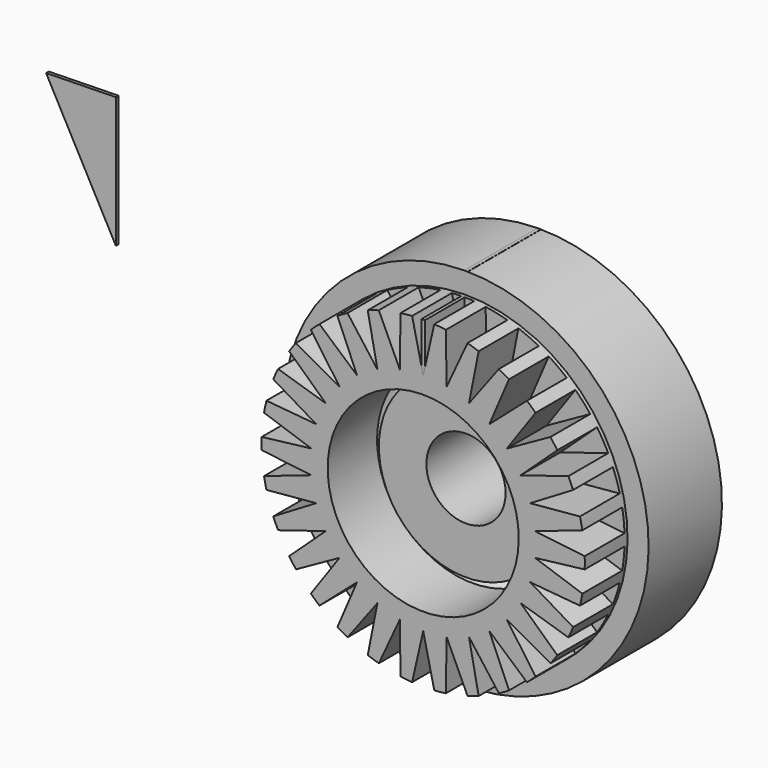
from build123d import *

# Parameters (mm, degrees)
F2_DEPTH = 0.5
F0_W     = 16.1312930286
F0_H     = 19.9230848044
F5_DEPTH = 15
F7_DEPTH = 1


with BuildPart() as f2:
    # F0 (on Right) → F2 (new body, symmetric)
    with BuildSketch(Plane.YZ):
        with BuildLine():
            Line((0, 16.1320931972), (0, 11.9378846139))
            Line((0, 11.9378846139), (13.8204824179, 11.9378846139))
            Line((13.8204824179, 11.9378846139), (13.8204824179, 26.2730848044))
            Line((13.8204824179, 26.2730848044), (11.3400983003, 26.2730848044))
            ThreePointArc((11.3400983003, 26.2730848044), (7.6065356805, 19.0371254581), (0, 16.1320931972))
        make_face()
        with BuildLine():
            Line((-13.8204824179, 11.9378846139), (0, 11.9378846139))
            Line((0, 11.9378846139), (0, 16.1320931972))
            ThreePointArc((0, 16.1320931972), (-7.6065356805, 19.0371254581), (-11.3400983003, 26.2730848044))
            Line((-11.3400983003, 26.2730848044), (-13.8204824179, 26.2730848044))
            Line((-13.8204824179, 26.2730848044), (-13.8204824179, 11.9378846139))
        make_face()
    extrude(amount=F2_DEPTH, both=True)


with BuildPart() as f2b:
    # F0 (on Right) → F2, piece 2 (new body, symmetric)
    with BuildSketch(Plane.YZ):
        with Locations((-21.8861289322, 38.7746272066)):
            Rectangle(F0_W, F0_H)
        with BuildLine():
            Line((-13.8204824179, 28.8130848044), (-11.3400983003, 28.8130848044))
            ThreePointArc((-11.3400983003, 28.8130848044), (0, 38.9540764116), (11.3400983003, 28.8130848044))
            Line((11.3400983003, 28.8130848044), (13.8204824179, 28.8130848044))
            Line((13.8204824179, 28.8130848044), (13.8204824179, 55.0861696088))
            Line((13.8204824179, 55.0861696088), (0, 55.0861696088))
            Line((0, 55.0861696088), (-13.8204824179, 55.0861696088))
            Line((-13.8204824179, 55.0861696088), (-13.8204824179, 48.7361696088))
            Line((-13.8204824179, 48.7361696088), (-13.8204824179, 28.8130848044))
        make_face()
    extrude(amount=F2_DEPTH, both=True)


with BuildPart() as f3:
    # F2_face (on face) → F3 (revolve)
    with BuildSketch(Plane(origin=(-0.5, -8.0664830441, 42.5658458946), x_dir=(0, 1, 0), z_dir=(-1, 0, 0))):
        with BuildLine():
            Line((-21.8852924024, -6.1703237142), (-5.7539993738, -6.1703237142))
            Line((-5.7539993738, -6.1703237142), (-5.7539993738, -12.5203237142))
            Line((-5.7539993738, -12.5203237142), (21.8869654621, -12.5203237142))
            Line((21.8869654621, -12.5203237142), (21.8869654621, 13.7527610902))
            Line((21.8869654621, 13.7527610902), (19.4065813444, 13.7527610902))
            ThreePointArc((19.4065813444, 13.7527610902), (8.0664830441, 3.611769483), (-3.2736152561, 13.7527610902))
            Line((-3.2736152561, 13.7527610902), (-21.8852924024, 13.7527610902))
            Line((-21.8852924024, 13.7527610902), (-21.8852924024, -6.1703237142))
        make_face()
    revolve(axis=Axis((0, -0.1056473702, 0), (0, -1, 0)))

    # F4 (on face) → F5 (cut)
    with BuildSketch(Plane.XZ.offset(29.9517754465)):
        with BuildLine():
            Line((-7.0547712791, 33.1900893753), (-6.8376785657, 48.2567133151))
            ThreePointArc((-6.8376785657, 48.2567133151), (-8.490521681, 47.9934919518), (-10.1333526715, 47.6736760883))
            ThreePointArc((-10.1333526715, 47.6736760883), (-11.7642342913, 47.2976428554), (-13.3812433852, 46.865835676))
            Line((-13.3812433852, 46.865835676), (-7.0547712791, 33.1900893753))
        make_face()
        with BuildLine():
            ThreePointArc((3.3448759751, 48.6238216603), (1.6734246487, 48.7099977221), (0, 48.7387343716))
            ThreePointArc((0, 48.7387343716), (-1.6734246487, 48.7099977221), (-3.3448759751, 48.6238216603))
            Line((-3.3448759751, 48.6238216603), (0, 33.9315757155))
            Line((0, 33.9315757155), (3.3448759751, 48.6238216603))
        make_face()
        with BuildLine():
            ThreePointArc((10.1333526715, 47.6736760883), (8.490521681, 47.9934919518), (6.8376785657, 48.2567133151))
            Line((6.8376785657, 48.2567133151), (7.0547712791, 33.1900893753))
            Line((7.0547712791, 33.1900893753), (13.3812433852, 46.865835676))
            ThreePointArc((13.3812433852, 46.865835676), (11.7642342913, 47.2976428554), (10.1333526715, 47.6736760883))
        make_face()
        with BuildLine():
            ThreePointArc((19.823829206, 44.5250493964), (18.2833914712, 45.1794402849), (16.7213937422, 45.7805550366))
            Line((16.7213937422, 45.7805550366), (13.8012152008, 30.9980368656))
            Line((13.8012152008, 30.9980368656), (22.832786249, 43.0595877854))
            ThreePointArc((22.832786249, 43.0595877854), (21.3408904443, 43.8181540367), (19.823829206, 44.5250493964))
        make_face()
        with BuildLine():
            ThreePointArc((28.647909279, 39.4304643909), (27.2771893206, 40.3908302825), (25.8743037741, 41.3035668235))
            Line((25.8743037741, 41.3035668235), (19.9444797926, 27.4512213998))
            Line((19.9444797926, 27.4512213998), (31.2864267899, 37.3714292858))
            ThreePointArc((31.2864267899, 37.3714292858), (29.9848472799, 38.4236016238), (28.647909279, 39.4304643909))
        make_face()
        with BuildLine():
            ThreePointArc((36.2199382485, 32.6125788832), (35.0788431063, 33.83694718), (33.8963825724, 35.0214145438))
            Line((33.8963825724, 35.0214145438), (25.2160749133, 22.7046558333))
            Line((25.2160749133, 22.7046558333), (38.3727003512, 30.0499599983))
            ThreePointArc((38.3727003512, 30.0499599983), (37.3183224061, 31.349753443), (36.2199382485, 32.6125788832))
        make_face()
        with BuildLine():
            ThreePointArc((42.2089821141, 24.3693671858), (41.3473831213, 25.8042271182), (40.4370267994, 27.2086583971))
            Line((40.4370267994, 27.2086583971), (29.3856065601, 16.9657878578))
            Line((29.3856065601, 16.9657878578), (43.7819027744, 21.4151632632))
            ThreePointArc((43.7819027744, 21.4151632632), (43.02080777, 22.9057706039), (42.2089821141, 24.3693671858))
        make_face()
        with BuildLine():
            ThreePointArc((46.35329092, 15.0610972051), (45.8088440871, 16.6437385088), (45.2103789168, 18.2067533168))
            Line((45.2103789168, 18.2067533168), (32.2708461924, 10.485433542))
            Line((32.2708461924, 10.485433542), (47.2776259576, 11.8444211322))
            ThreePointArc((47.2776259576, 11.8444211322), (46.8430773976, 13.4606956754), (46.35329092, 15.0610972051))
        make_face()
        with BuildLine():
            ThreePointArc((48.471738485, 5.0945850055), (48.268238751, 6.7558386611), (48.0078205322, 8.4091257508))
            Line((48.0078205322, 8.4091257508), (33.7456949935, 3.5468154658))
            Line((33.7456949935, 3.5468154658), (48.7070900231, 1.7560209619))
            ThreePointArc((48.7070900231, 1.7560209619), (48.6180797649, 3.4273237543), (48.471738485, 5.0945850055))
        make_face()
        with BuildLine():
            ThreePointArc((48.471738485, -5.0945850055), (48.6180797649, -3.4273237543), (48.7070900231, -1.7560209619))
            Line((48.7070900231, -1.7560209619), (33.7456949935, -3.5468154658))
            Line((33.7456949935, -3.5468154658), (48.0078205322, -8.4091257508))
            ThreePointArc((48.0078205322, -8.4091257508), (48.268238751, -6.7558386611), (48.471738485, -5.0945850055))
        make_face()
        with BuildLine():
            ThreePointArc((46.35329092, -15.0610972051), (46.8430773976, -13.4606956754), (47.2776259576, -11.8444211322))
            Line((47.2776259576, -11.8444211322), (32.2708461924, -10.485433542))
            Line((32.2708461924, -10.485433542), (45.2103789168, -18.2067533168))
            ThreePointArc((45.2103789168, -18.2067533168), (45.8088440871, -16.6437385088), (46.35329092, -15.0610972051))
        make_face()
        with BuildLine():
            ThreePointArc((42.2089821141, -24.3693671858), (43.02080777, -22.9057706039), (43.7819027744, -21.4151632632))
            Line((43.7819027744, -21.4151632632), (29.3856065601, -16.9657878578))
            Line((29.3856065601, -16.9657878578), (40.4370267994, -27.2086583971))
            ThreePointArc((40.4370267994, -27.2086583971), (41.3473831213, -25.8042271182), (42.2089821141, -24.3693671858))
        make_face()
        with BuildLine():
            ThreePointArc((36.2199382485, -32.6125788832), (37.3183224061, -31.349753443), (38.3727003512, -30.0499599983))
            Line((38.3727003512, -30.0499599983), (25.2160749133, -22.7046558333))
            Line((25.2160749133, -22.7046558333), (33.8963825724, -35.0214145438))
            ThreePointArc((33.8963825724, -35.0214145438), (35.0788431063, -33.83694718), (36.2199382485, -32.6125788832))
        make_face()
        with BuildLine():
            ThreePointArc((28.647909279, -39.4304643909), (29.9848472799, -38.4236016238), (31.2864267899, -37.3714292858))
            Line((31.2864267899, -37.3714292858), (19.9444797926, -27.4512213998))
            Line((19.9444797926, -27.4512213998), (25.8743037741, -41.3035668235))
            ThreePointArc((25.8743037741, -41.3035668235), (27.2771893206, -40.3908302825), (28.647909279, -39.4304643909))
        make_face()
        with BuildLine():
            ThreePointArc((19.823829206, -44.5250493964), (21.3408904443, -43.8181540367), (22.832786249, -43.0595877854))
            Line((22.832786249, -43.0595877854), (13.8012152008, -30.9980368656))
            Line((13.8012152008, -30.9980368656), (16.7213937422, -45.7805550366))
            ThreePointArc((16.7213937422, -45.7805550366), (18.2833914712, -45.1794402849), (19.823829206, -44.5250493964))
        make_face()
        with BuildLine():
            ThreePointArc((10.1333526715, -47.6736760883), (11.7642342913, -47.2976428554), (13.3812433852, -46.865835676))
            Line((13.3812433852, -46.865835676), (7.0547712791, -33.1900893753))
            Line((7.0547712791, -33.1900893753), (6.8376785657, -48.2567133151))
            ThreePointArc((6.8376785657, -48.2567133151), (8.490521681, -47.9934919518), (10.1333526715, -47.6736760883))
        make_face()
        with BuildLine():
            Line((0, -33.9315757155), (-3.3448759751, -48.6238216603))
            ThreePointArc((-3.3448759751, -48.6238216603), (-1.6734246487, -48.7099977221), (0, -48.7387343716))
            ThreePointArc((0, -48.7387343716), (1.6734246487, -48.7099977221), (3.3448759751, -48.6238216603))
            Line((3.3448759751, -48.6238216603), (0, -33.9315757155))
        make_face()
        with BuildLine():
            Line((-7.0547712791, -33.1900893753), (-13.3812433852, -46.865835676))
            ThreePointArc((-13.3812433852, -46.865835676), (-11.7642342913, -47.2976428554), (-10.1333526715, -47.6736760883))
            ThreePointArc((-10.1333526715, -47.6736760883), (-8.490521681, -47.9934919518), (-6.8376785657, -48.2567133151))
            Line((-6.8376785657, -48.2567133151), (-7.0547712791, -33.1900893753))
        make_face()
        with BuildLine():
            Line((-13.8012152008, -30.9980368656), (-22.832786249, -43.0595877854))
            ThreePointArc((-22.832786249, -43.0595877854), (-21.3408904443, -43.8181540367), (-19.823829206, -44.5250493964))
            ThreePointArc((-19.823829206, -44.5250493964), (-18.2833914712, -45.1794402849), (-16.7213937422, -45.7805550366))
            Line((-16.7213937422, -45.7805550366), (-13.8012152008, -30.9980368656))
        make_face()
        with BuildLine():
            Line((-19.9444797926, -27.4512213998), (-31.2864267899, -37.3714292858))
            ThreePointArc((-31.2864267899, -37.3714292858), (-29.9848472799, -38.4236016238), (-28.647909279, -39.4304643909))
            ThreePointArc((-28.647909279, -39.4304643909), (-27.2771893206, -40.3908302825), (-25.8743037741, -41.3035668235))
            Line((-25.8743037741, -41.3035668235), (-19.9444797926, -27.4512213998))
        make_face()
        with BuildLine():
            Line((-25.2160749133, -22.7046558333), (-38.3727003512, -30.0499599983))
            ThreePointArc((-38.3727003512, -30.0499599983), (-37.3183224061, -31.349753443), (-36.2199382485, -32.6125788832))
            ThreePointArc((-36.2199382485, -32.6125788832), (-35.0788431063, -33.83694718), (-33.8963825724, -35.0214145438))
            Line((-33.8963825724, -35.0214145438), (-25.2160749133, -22.7046558333))
        make_face()
        with BuildLine():
            Line((-29.3856065601, -16.9657878578), (-43.7819027744, -21.4151632632))
            ThreePointArc((-43.7819027744, -21.4151632632), (-43.02080777, -22.9057706039), (-42.2089821141, -24.3693671858))
            ThreePointArc((-42.2089821141, -24.3693671858), (-41.3473831213, -25.8042271182), (-40.4370267994, -27.2086583971))
            Line((-40.4370267994, -27.2086583971), (-29.3856065601, -16.9657878578))
        make_face()
        with BuildLine():
            Line((-32.2708461924, -10.485433542), (-47.2776259576, -11.8444211322))
            ThreePointArc((-47.2776259576, -11.8444211322), (-46.8430773976, -13.4606956754), (-46.35329092, -15.0610972051))
            ThreePointArc((-46.35329092, -15.0610972051), (-45.8088440871, -16.6437385088), (-45.2103789168, -18.2067533168))
            Line((-45.2103789168, -18.2067533168), (-32.2708461924, -10.485433542))
        make_face()
        with BuildLine():
            Line((-33.7456949935, -3.5468154658), (-48.7070900231, -1.7560209619))
            ThreePointArc((-48.7070900231, -1.7560209619), (-48.6180797649, -3.4273237543), (-48.471738485, -5.0945850055))
            ThreePointArc((-48.471738485, -5.0945850055), (-48.268238751, -6.7558386611), (-48.0078205322, -8.4091257508))
            Line((-48.0078205322, -8.4091257508), (-33.7456949935, -3.5468154658))
        make_face()
        with BuildLine():
            Line((-33.7456949935, 3.5468154658), (-48.0078205322, 8.4091257508))
            ThreePointArc((-48.0078205322, 8.4091257508), (-48.268238751, 6.7558386611), (-48.471738485, 5.0945850055))
            ThreePointArc((-48.471738485, 5.0945850055), (-48.6180797649, 3.4273237543), (-48.7070900231, 1.7560209619))
            Line((-48.7070900231, 1.7560209619), (-33.7456949935, 3.5468154658))
        make_face()
        with BuildLine():
            Line((-32.2708461924, 10.485433542), (-45.2103789168, 18.2067533168))
            ThreePointArc((-45.2103789168, 18.2067533168), (-45.8088440871, 16.6437385088), (-46.35329092, 15.0610972051))
            ThreePointArc((-46.35329092, 15.0610972051), (-46.8430773976, 13.4606956754), (-47.2776259576, 11.8444211322))
            Line((-47.2776259576, 11.8444211322), (-32.2708461924, 10.485433542))
        make_face()
        with BuildLine():
            Line((-29.3856065601, 16.9657878578), (-40.4370267994, 27.2086583971))
            ThreePointArc((-40.4370267994, 27.2086583971), (-41.3473831213, 25.8042271182), (-42.2089821141, 24.3693671858))
            ThreePointArc((-42.2089821141, 24.3693671858), (-43.02080777, 22.9057706039), (-43.7819027744, 21.4151632632))
            Line((-43.7819027744, 21.4151632632), (-29.3856065601, 16.9657878578))
        make_face()
        with BuildLine():
            Line((-25.2160749133, 22.7046558333), (-33.8963825724, 35.0214145438))
            ThreePointArc((-33.8963825724, 35.0214145438), (-35.0788431063, 33.83694718), (-36.2199382485, 32.6125788832))
            ThreePointArc((-36.2199382485, 32.6125788832), (-37.3183224061, 31.349753443), (-38.3727003512, 30.0499599983))
            Line((-38.3727003512, 30.0499599983), (-25.2160749133, 22.7046558333))
        make_face()
        with BuildLine():
            Line((-19.9444797926, 27.4512213998), (-25.8743037741, 41.3035668235))
            ThreePointArc((-25.8743037741, 41.3035668235), (-27.2771893206, 40.3908302825), (-28.647909279, 39.4304643909))
            ThreePointArc((-28.647909279, 39.4304643909), (-29.9848472799, 38.4236016238), (-31.2864267899, 37.3714292858))
            Line((-31.2864267899, 37.3714292858), (-19.9444797926, 27.4512213998))
        make_face()
        with BuildLine():
            Line((-13.8012152008, 30.9980368656), (-16.7213937422, 45.7805550366))
            ThreePointArc((-16.7213937422, 45.7805550366), (-18.2833914712, 45.1794402849), (-19.823829206, 44.5250493964))
            ThreePointArc((-19.823829206, 44.5250493964), (-21.3408904443, 43.8181540367), (-22.832786249, 43.0595877854))
            Line((-22.832786249, 43.0595877854), (-13.8012152008, 30.9980368656))
        make_face()
    extrude(amount=-F5_DEPTH, mode=Mode.SUBTRACT)


with BuildPart() as f3b:
    # F2_face (on face) → F3, piece 2 (revolve)
    with BuildSketch(Plane(origin=(-0.5, -8.0664830441, 42.5658458946), x_dir=(0, 1, 0), z_dir=(-1, 0, 0))):
        with BuildLine():
            Line((21.8869654621, 16.2927610902), (21.8869654621, 30.6279612808))
            Line((21.8869654621, 30.6279612808), (-5.7539993738, 30.6279612808))
            Line((-5.7539993738, 30.6279612808), (-5.7539993738, 16.2927610902))
            Line((-5.7539993738, 16.2927610902), (-3.2736152561, 16.2927610902))
            ThreePointArc((-3.2736152561, 16.2927610902), (8.0664830441, 26.4337526974), (19.4065813444, 16.2927610902))
            Line((19.4065813444, 16.2927610902), (21.8869654621, 16.2927610902))
        make_face()
    revolve(axis=Axis((0, -0.1056473702, 0), (0, -1, 0)))


with BuildPart() as f7:
    # F6 (on Front) → F7 (new body)
    with BuildSketch(Plane.XZ):
        Polygon((-115.843527019, 58.3605729043), (-136.9059830904, 57.9217672348), (-115.843527019, 18.8684556633), align=None)
    extrude(amount=F7_DEPTH)


solid = Compound([f2.part, f2b.part, f3.part, f3b.part, f7.part])
